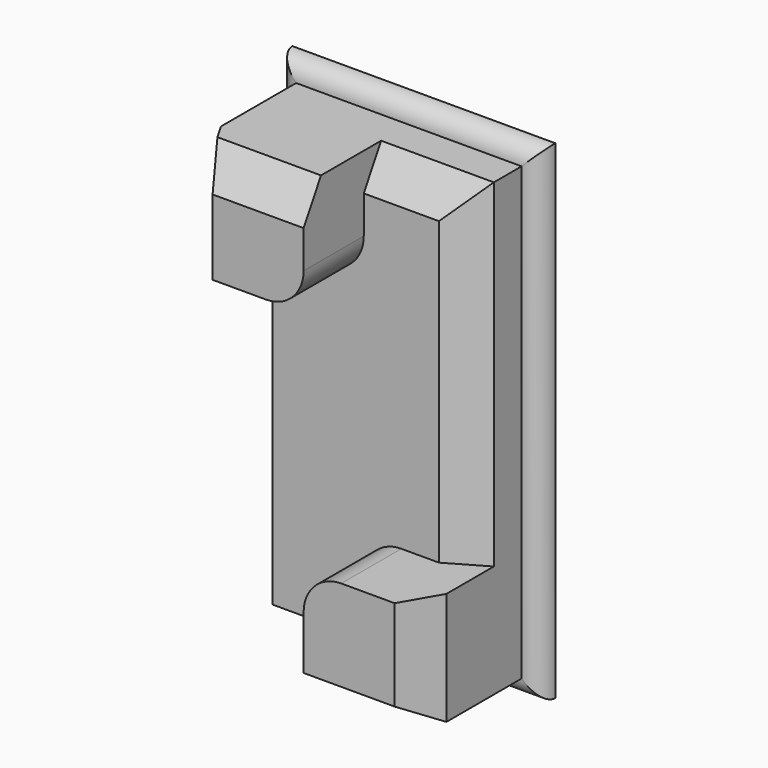
from build123d import *

# Parameters (mm, degrees)
F0_W        = 88.9
F0_H        = 165.1
F1_DEPTH    = 6.35
F2_DEPTH    = 25.4
F3_DEPTH    = 50.8
F4_R        = 6.34999
F5_C1_SIZE2 = 7.3323484187
F5_C1_SIZE  = 12.7
F5_C2_SIZE2 = 7.3323484187
F5_C2_SIZE  = 12.7
F5_C3_SIZE2 = 12.7
F5_C3_SIZE  = 7.3323484187
F5_C4_SIZE2 = 12.7
F5_C4_SIZE  = 7.3323484187
F5_C5_SIZE2 = 7.3323484187
F5_C5_SIZE  = 12.7
F5_C6_SIZE2 = 12.7
F5_C6_SIZE  = 7.3323484187
F5_C7_SIZE2 = 7.3323484187
F5_C7_SIZE  = 12.7
F5_C8_SIZE2 = 7.3323484187
F5_C8_SIZE  = 12.7


# Not quite as in the source:
# - a fillet or chamfer is up to 0.001 mm smaller than in the source, because OpenCascade refuses the exact size


with BuildPart() as f1:
    # F0 (on Front) → F1 (new body)
    with BuildSketch(Plane.XZ):
        with Locations((8.2040027817, 0.7496795987)):
            Rectangle(F0_W, F0_H)
        Polygon((-29.8959972183, 38.8496795987), (-29.8959972183, 76.9496795987), (8.2040027817, 76.9496795987), (46.3040027817, 76.9496795987), (46.3040027817, -37.3503204013), (46.3040027817, -75.4503204013), (8.2040027817, -75.4503204013), (-29.8959972183, -75.4503204013), align=None, mode=Mode.SUBTRACT)
    extrude(amount=F1_DEPTH)

    # F0 (on Front) → F2 (join)
    with BuildSketch(Plane.XZ):
        with BuildLine():
            Line((46.3040027817, 76.9496795987), (8.2040027817, 76.9496795987))
            Line((8.2040027817, 76.9496795987), (8.2040027817, 51.5496795987))
            ThreePointArc((8.2040027817, 51.5496795987), (4.4842589027, 42.5694234776), (-4.4959972183, 38.8496795987))
            Line((-4.4959972183, 38.8496795987), (-29.8959972183, 38.8496795987))
            Line((-29.8959972183, 38.8496795987), (-29.8959972183, -75.4503204013))
            Line((-29.8959972183, -75.4503204013), (8.2040027817, -75.4503204013))
            Line((8.2040027817, -75.4503204013), (8.2040027817, -50.0503204013))
            ThreePointArc((8.2040027817, -50.0503204013), (11.9237466606, -41.0700642803), (20.9040027817, -37.3503204013))
            Line((20.9040027817, -37.3503204013), (46.3040027817, -37.3503204013))
            Line((46.3040027817, -37.3503204013), (46.3040027817, 76.9496795987))
        make_face()
    extrude(amount=F2_DEPTH)

    # F0 (on Front) → F3 (join)
    with BuildSketch(Plane.XZ):
        with BuildLine():
            Line((8.2040027817, 76.9496795987), (-29.8959972183, 76.9496795987))
            Line((-29.8959972183, 76.9496795987), (-29.8959972183, 38.8496795987))
            Line((-29.8959972183, 38.8496795987), (-4.4959972183, 38.8496795987))
            ThreePointArc((-4.4959972183, 38.8496795987), (4.4842589027, 42.5694234776), (8.2040027817, 51.5496795987))
            Line((8.2040027817, 51.5496795987), (8.2040027817, 76.9496795987))
        make_face()
        with BuildLine():
            Line((46.3040027817, -75.4503204013), (46.3040027817, -37.3503204013))
            Line((46.3040027817, -37.3503204013), (20.9040027817, -37.3503204013))
            ThreePointArc((20.9040027817, -37.3503204013), (11.9237466606, -41.0700642803), (8.2040027817, -50.0503204013))
            Line((8.2040027817, -50.0503204013), (8.2040027817, -75.4503204013))
            Line((8.2040027817, -75.4503204013), (46.3040027817, -75.4503204013))
        make_face()
    extrude(amount=F3_DEPTH)

    # F4 (radius 6.35 in the source; OpenCascade refuses exactly that, so slightly less here)
    f4_edges = [f1.edges().sort_by_distance(p)[0] for p in [
        (8.204003, -6.35, 83.29968),
        (-36.245997, -6.35, 0.74968),
        (8.204003, -6.35, -81.80032),
        (52.654003, -6.35, 0.74968),
    ]]
    fillet(f4_edges, radius=F4_R)

    # F5: chamfer of 12.7 x 7.3323484187 on 8 edges, made by hand

    # F5_c1
    f5_c1_edges = [f1.edges().sort_by_distance(p)[0] for p in [
        (-29.8959972183, -50.8, 57.8996795987),
    ]]
    f5_c1_side = f1.faces().sort_by_distance((-29.8959972183, -50.6533530316, 57.8996795987))[0]
    chamfer(f5_c1_edges, length=F5_C1_SIZE, length2=F5_C1_SIZE2, reference=f5_c1_side)

    # F5_c2
    f5_c2_edges = [f1.edges().sort_by_distance(p)[0] for p in [
        (-29.8959972183, -25.4, -18.3003204013),
    ]]
    f5_c2_side = f1.faces().sort_by_distance((-29.8959972183, -25.2533530316, -18.3003204013))[0]
    chamfer(f5_c2_edges, length=F5_C2_SIZE, length2=F5_C2_SIZE2, reference=f5_c2_side)

    # F5_c3
    f5_c3_edges = [f1.edges().sort_by_distance(p)[0] for p in [
        (27.2540027817, -25.4, 76.9496795987),
    ]]
    f5_c3_side = f1.faces().sort_by_distance((27.2540027817, -25.2533530316, 76.9496795987))[0]
    chamfer(f5_c3_edges, length=F5_C3_SIZE, length2=F5_C3_SIZE2, reference=f5_c3_side)

    # F5_c4
    f5_c4_edges = [f1.edges().sort_by_distance(p)[0] for p in [
        (-7.179823009, -50.8, 76.9496795987),
    ]]
    f5_c4_side = f1.faces().sort_by_distance((-7.179823009, -50.6533530316, 76.9496795987))[0]
    chamfer(f5_c4_edges, length=F5_C4_SIZE, length2=F5_C4_SIZE2, reference=f5_c4_side)

    # F5_c5
    f5_c5_edges = [f1.edges().sort_by_distance(p)[0] for p in [
        (46.3040027817, -50.8, -56.4003204013),
    ]]
    f5_c5_side = f1.faces().sort_by_distance((46.3040027817, -50.6533530316, -56.4003204013))[0]
    chamfer(f5_c5_edges, length=F5_C5_SIZE, length2=F5_C5_SIZE2, reference=f5_c5_side)

    # F5_c6
    f5_c6_edges = [f1.edges().sort_by_distance(p)[0] for p in [
        (46.3040027817, -25.4, 13.4496795987),
    ]]
    f5_c6_side = f1.faces().sort_by_distance((46.3040027817, -25.2533530316, 13.4496795987))[0]
    chamfer(f5_c6_edges, length=F5_C6_SIZE, length2=F5_C6_SIZE2, reference=f5_c6_side)

    # F5_c7
    f5_c7_edges = [f1.edges().sort_by_distance(p)[0] for p in [
        (-7.179823009, -25.4, -75.4503204013),
    ]]
    f5_c7_side = f1.faces().sort_by_distance((-7.179823009, -25.2533530316, -75.4503204013))[0]
    chamfer(f5_c7_edges, length=F5_C7_SIZE, length2=F5_C7_SIZE2, reference=f5_c7_side)

    # F5_c8
    f5_c8_edges = [f1.edges().sort_by_distance(p)[0] for p in [
        (23.5878285723, -50.8, -75.4503204013),
    ]]
    f5_c8_side = f1.faces().sort_by_distance((23.5878285723, -50.6533530316, -75.4503204013))[0]
    chamfer(f5_c8_edges, length=F5_C8_SIZE, length2=F5_C8_SIZE2, reference=f5_c8_side)


solid = f1.part
